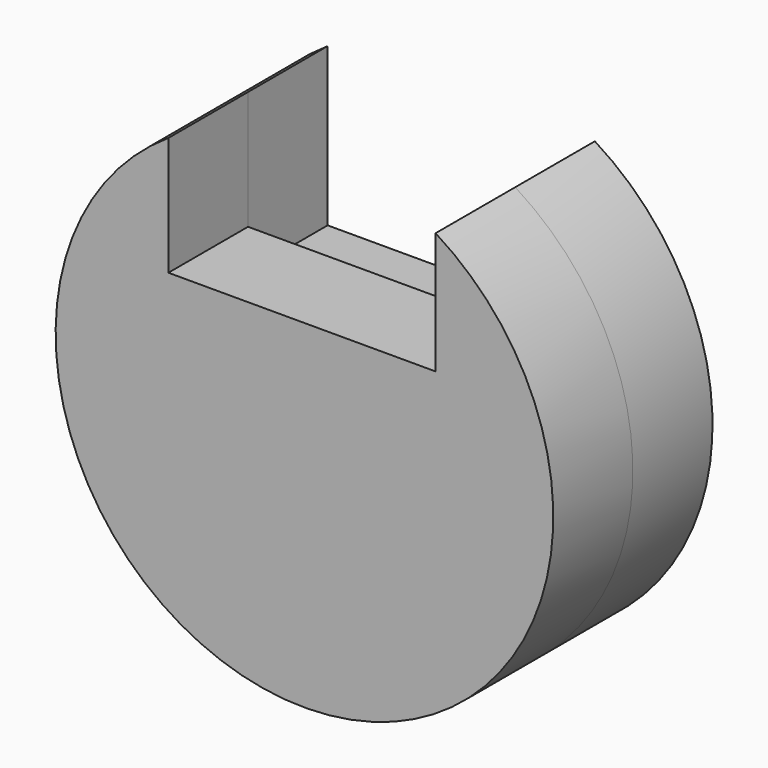
from build123d import *

# Parameters (mm, degrees)
F0_R     = 63.5
F1_DEPTH = 25.4
F2_DEPTH = 25.4
F4_DEPTH = 50.8
F5_W     = 68.1968787685
F5_H     = 50
F6_DEPTH = 64.06949


with BuildPart() as f1:
    # F0 (on Front) → F1 (new body)
    with BuildSketch(Plane.XZ):
        with Locations((-41.5502935648, 45.182749629)):
            Circle(F0_R)
    extrude(amount=F1_DEPTH)


with BuildPart() as f2:
    # F2 (new): a face of the model
    f2_faces = [f1.part.faces().sort_by_distance(p)[0] for p in [
        (-41.5502935648, -25.4, 45.182749629),
    ]]
    extrude(f2_faces, amount=F2_DEPTH)

    # F5 (on face) → F6 (cut)
    with BuildSketch(Plane(origin=(0, -25.4, 0), x_dir=(-1, 0, 0), z_dir=(0, 1, 0))):
        with Locations((42.1763206832, 93.0761879683)):
            Rectangle(F5_W, F5_H)
    extrude(amount=-F6_DEPTH, mode=Mode.SUBTRACT)


with BuildPart() as f1_1:
    add(f1.part)

    # F3 (on face) → F4 (cut)
    with BuildSketch(Plane(origin=(0, 0, 0), x_dir=(-1, 0, 0), z_dir=(0, 1, 0))):
        with BuildLine():
            ThreePointArc((76.2747600675, 98.3472248555), (42.2924103642, 108.6784129664), (8.077881299, 99.144287942))
            Line((8.077881299, 99.144287942), (8.077881299, 58.0761879683))
            Line((8.077881299, 58.0761879683), (76.2747600675, 58.0761879683))
            Line((76.2747600675, 58.0761879683), (76.2747600675, 98.3472248555))
        make_face()
    extrude(amount=-F4_DEPTH, mode=Mode.SUBTRACT)


solid = Compound([f2.part, f1_1.part])
